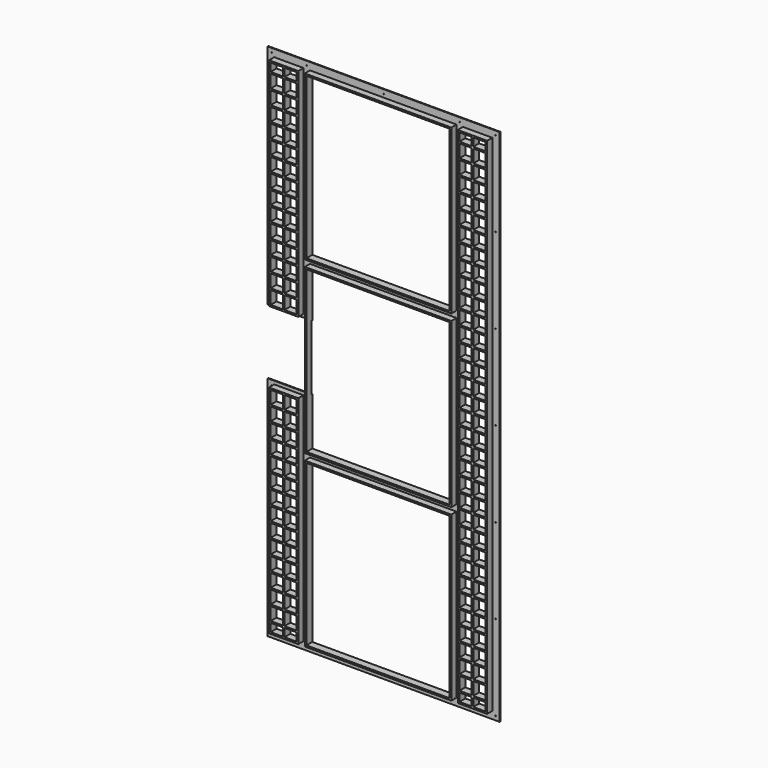
from build123d import *

# Parameters (mm, degrees)
F0_W      = 114.3
F0_H      = 844.55
F0_H_2    = 1968.5
F0_W_2    = 571.5
F0_H_3    = 25.4
F1_DEPTH  = 3.175
F2_W      = 114.3
F2_H      = 1968.5
F2_W_2    = 101.6000261307
F2_H_2    = 1955.8000261307
F2_W_3    = 571.5
F2_H_3    = 638.96875
F2_W_4    = 558.8
F2_H_4    = 626.26875
F2_H_5    = 639.7625
F2_H_6    = 627.0625
F2_H_7    = 844.55
F2_W_5    = 101.6000169754
F2_H_8    = 831.8500169754
F2_W_6    = 101.5999731064
F2_H_9    = 831.8499731064
F2_W_7    = 558.8000261307
F2_H_10   = 626.2687761307
F3_DEPTH  = 28.575
F4_W      = 47.6250084877
F4_H      = 6.35
F4_W_2    = 6.35
F4_H_2    = 50.8
F4_H_3    = 6.3500062943
F4_H_4    = 6.3500309944
F4_H_5    = 31.75
F4_H_6    = 6.3500188828
F4_H_7    = 6.3500125885
F5_DEPTH  = 28.575
F4_H_8    = 6.3500052452
F4_W_3    = 47.6249865532
F4_H_9    = 6.3499976873
F4_H_10   = 6.3499988437
F4_H_11   = 6.349999775
F4_H_12   = 6.349996756
F4_H_13   = 31.7498180389
F6_DEPTH  = 28.575
F4_H_14   = 31.7500045776
F4_W_4    = 47.6250130653
F7_DEPTH  = 28.575
F4_H_15   = 31.7498445511
F8_DEPTH  = 28.575
F9_DEPTH  = 28.575
F10_R     = 1.5875
F11_DEPTH = 25.4
F10_R_2   = 4.7625
F12_DEPTH = 1.5875
F13_W     = 19.05
F13_H     = 254
F14_DEPTH = 3.175


# Not quite as in the source:
# - ends of sketch curves that miss each other by under 0.0002 mm in the source are joined


with BuildPart() as f1:
    # F0 (on Front) → F1 (new body)
    with BuildSketch(Plane.XZ):
        Polygon((-450.85, -1508.125), (450.85, -1508.125), (450.85, 511.175), (-450.85, 511.175), (-450.85, -371.475), (-298.45, -371.475), (-298.45, -625.475), (-450.85, -625.475), align=None)
        with Locations((-368.3, -1060.45)):
            Rectangle(F0_W, F0_H, mode=Mode.SUBTRACT)
        Polygon((-285.75, -153.19375), (-285.75, 485.775), (285.75, 485.775), (285.75, -153.19375), (285.75, -178.59375), (285.75, -818.35625), (285.75, -843.75625), (285.75, -1482.725), (-285.75, -1482.725), (-285.75, -843.75625), (-285.75, -818.35625), (-285.75, -178.59375), align=None, mode=Mode.SUBTRACT)
        with Locations((-368.3, 63.5)):
            Rectangle(F0_W, F0_H, mode=Mode.SUBTRACT)
        with Locations((368.3, -498.475)):
            Rectangle(F0_W, F0_H_2, mode=Mode.SUBTRACT)
        Polygon((450.85, 511.175), (450.85, -1508.125), (-450.85, -1508.125), (-450.8499999999, -1511.3), (454.025, -1511.3), (454.025, 514.35), (-450.85, 514.35), (-450.85, 511.175), align=None)
        with Locations((0, -831.05625)):
            Rectangle(F0_W_2, F0_H_3)
        with Locations((0, -165.89375)):
            Rectangle(F0_W_2, F0_H_3)
    extrude(amount=F1_DEPTH)

    # F2 (on Front) → F3 (join)
    with BuildSketch(Plane.XZ):
        with Locations((368.3, -498.475)):
            Rectangle(F2_W, F2_H)
        with Locations((368.3, -498.475)):
            Rectangle(F2_W_2, F2_H_2, mode=Mode.SUBTRACT)
        with Locations((0, -1163.240625)):
            Rectangle(F2_W_3, F2_H_3)
        with Locations((0, -1163.240625)):
            Rectangle(F2_W_4, F2_H_4, mode=Mode.SUBTRACT)
        with Locations((0, -498.475)):
            Rectangle(F2_W_3, F2_H_5)
        with Locations((0, -498.475)):
            Rectangle(F2_W_4, F2_H_6, mode=Mode.SUBTRACT)
        with Locations((-368.3, -1060.45)):
            Rectangle(F2_W, F2_H_7)
        with Locations((-368.3, -1060.45)):
            Rectangle(F2_W_5, F2_H_8, mode=Mode.SUBTRACT)
        with Locations((-368.3, 63.5)):
            Rectangle(F2_W, F2_H_7)
        with Locations((-368.3, 63.5)):
            Rectangle(F2_W_6, F2_H_9, mode=Mode.SUBTRACT)
        with Locations((0, 166.290625)):
            Rectangle(F2_W_3, F2_H_3)
        with Locations((0, 166.290625)):
            Rectangle(F2_W_7, F2_H_10, mode=Mode.SUBTRACT)
    extrude(amount=F3_DEPTH)

    # F4 (on Front) → F5 (join)
    with BuildSketch(Plane.XZ):
        with Locations((-341.3124957561, -1098.5499523163)):
            Rectangle(F4_W, F4_H)
        with Locations((-368.3, -1098.5499523163)):
            Rectangle(F4_W_2, F4_H)
        with Locations((-395.2875042439, -1098.5499523163)):
            Rectangle(F4_W, F4_H)
        with Locations((-368.3, -1127.1249523163)):
            Rectangle(F4_W_2, F4_H_2)
        with Locations((-395.2875042439, -1155.6999523163)):
            Rectangle(F4_W, F4_H)
        with Locations((-368.3, -1155.6999523163)):
            Rectangle(F4_W_2, F4_H)
        with Locations((-341.3124957561, -1155.6999523163)):
            Rectangle(F4_W, F4_H)
        with Locations((-395.2875042439, -1212.8499554634)):
            Rectangle(F4_W, F4_H_3)
        with Locations((-368.3, -1212.8499554634)):
            Rectangle(F4_W_2, F4_H_3)
        with Locations((-341.3124957561, -1212.8499554634)):
            Rectangle(F4_W, F4_H_3)
        with Locations((-368.3, -1241.4249586105)):
            Rectangle(F4_W_2, F4_H_2)
        with Locations((-368.3, -1269.9999617577)):
            Rectangle(F4_W_2, F4_H_3)
        with Locations((-395.2875042439, -1269.9999617577)):
            Rectangle(F4_W, F4_H_3)
        with Locations((-341.3124957561, -1269.9999617577)):
            Rectangle(F4_W, F4_H_3)
        Polygon((-317.4999915123, -1330.324971199), (-317.4999915123, -1323.9749649048), (-365.125, -1323.9749649048), (-371.475, -1323.9749649048), (-419.1000084877, -1323.9749649048), (-419.1000084877, -1330.324971199), (-371.475, -1330.324971199), (-365.125, -1330.324971199), align=None)
        with Locations((-368.3, -1355.724971199)):
            Rectangle(F4_W_2, F4_H_2)
        Polygon((-317.4999915123, -1387.4749774933), (-317.4999915123, -1381.124971199), (-365.125, -1381.124971199), (-371.475, -1381.124971199), (-419.1000084877, -1381.124971199), (-419.1000084877, -1387.4749774933), (-371.475, -1387.4749774933), (-365.125, -1387.4749774933), align=None)
        with Locations((-395.2875042439, -1441.4499929905)):
            Rectangle(F4_W, F4_H_4)
        with Locations((-341.3124957561, -1441.4499929905)):
            Rectangle(F4_W, F4_H_4)
        with Locations((-368.3, -1441.4499929905)):
            Rectangle(F4_W_2, F4_H_4)
        with Locations((-368.3, -1460.5000084877)):
            Rectangle(F4_W_2, F4_H_5)
        with Locations((-368.3, -1041.3999428749)):
            Rectangle(F4_W_2, F4_H_6)
        with Locations((-395.2875042439, -1041.3999428749)):
            Rectangle(F4_W, F4_H_6)
        with Locations((-341.3124957561, -1041.3999428749)):
            Rectangle(F4_W, F4_H_6)
        with Locations((-368.3, -1012.8249334335)):
            Rectangle(F4_W_2, F4_H_2)
        with Locations((-395.2875042439, -984.2499302864)):
            Rectangle(F4_W, F4_H_3)
        with Locations((-368.3, -984.2499302864)):
            Rectangle(F4_W_2, F4_H_3)
        with Locations((-341.3124957561, -984.2499302864)):
            Rectangle(F4_W, F4_H_3)
        with Locations((-341.3124957561, -869.949920845)):
            Rectangle(F4_W, F4_H)
        with Locations((-395.2875042439, -869.949920845)):
            Rectangle(F4_W, F4_H)
        with Locations((-368.3, -869.949920845)):
            Rectangle(F4_W_2, F4_H)
        with Locations((-368.3, -927.0999239922)):
            Rectangle(F4_W_2, F4_H_3)
        with Locations((-341.3124957561, -927.0999239922)):
            Rectangle(F4_W, F4_H_3)
        with Locations((-368.3, -898.524920845)):
            Rectangle(F4_W_2, F4_H_2)
        with Locations((-395.2875042439, -927.0999239922)):
            Rectangle(F4_W, F4_H_3)
        with Locations((-368.3, -812.7999145508)):
            Rectangle(F4_W_2, F4_H_7)
        with Locations((-395.2875042439, -812.7999145508)):
            Rectangle(F4_W, F4_H_7)
        with Locations((-341.3124957561, -812.7999145508)):
            Rectangle(F4_W, F4_H_7)
        with Locations((-368.3, -784.2249082565)):
            Rectangle(F4_W_2, F4_H_2)
        with Locations((-368.3, -755.6499082565)):
            Rectangle(F4_W_2, F4_H)
        with Locations((-395.2875042439, -755.6499082565)):
            Rectangle(F4_W, F4_H)
        with Locations((-341.3124957561, -755.6499082565)):
            Rectangle(F4_W, F4_H)
        Polygon((-317.4999915123, -701.6749082565), (-317.4999915123, -695.324895668), (-365.125, -695.324895668), (-371.475, -695.324895668), (-419.1000084877, -695.324895668), (-419.1000084877, -701.6749082565), (-371.475, -701.6749082565), (-365.125, -701.6749082565), align=None)
        Polygon((-365.125, -695.324895668), (-365.125, -644.5249435902), (-371.475, -644.5249915123), (-371.475, -695.324895668), align=None)
    extrude(amount=F5_DEPTH)

    # F4 (on Front) → F6 (join)
    with BuildSketch(Plane.XZ):
        with Locations((-368.3, -327.0248589516)):
            Rectangle(F4_W_2, F4_H_2)
        with Locations((-368.3, -298.449856329)):
            Rectangle(F4_W_2, F4_H_8)
        Polygon((-371.475, -301.6248589516), (-371.475, -295.2748537064), (-419.1000084877, -295.2748537064), (-419.0999865532, -301.6248589516), align=None)
        with Locations((-341.3125067234, -298.449856329)):
            Rectangle(F4_W_3, F4_H_8)
        with Locations((-341.3125067234, -241.2998537064)):
            Rectangle(F4_W_3, F4_H)
        with Locations((-368.3, -241.2998537064)):
            Rectangle(F4_W_2, F4_H)
        Polygon((-371.475, -244.4748537064), (-371.475, -238.1248537064), (-419.1000084877, -238.1248537064), (-419.0999865532, -244.4748537064), align=None)
        with Locations((-368.3, -212.7248537064)):
            Rectangle(F4_W_2, F4_H_2)
        with Locations((-368.3, -184.1498548627)):
            Rectangle(F4_W_2, F4_H_9)
        with Locations((-395.2875042439, -184.1498548627)):
            Rectangle(F4_W, F4_H_9)
        with Locations((-341.3125067234, -184.1498548627)):
            Rectangle(F4_W_3, F4_H_9)
        with Locations((-395.2875042439, -126.9998565972)):
            Rectangle(F4_W, F4_H_10)
        with Locations((-341.3125067234, -126.9998565972)):
            Rectangle(F4_W_3, F4_H_10)
        with Locations((-368.3, -98.4248571754)):
            Rectangle(F4_W_2, F4_H_2)
        with Locations((-368.3, -126.9998565972)):
            Rectangle(F4_W_2, F4_H_10)
        with Locations((-368.3, -69.8498577535)):
            Rectangle(F4_W_2, F4_H_10)
        with Locations((-395.2875042439, -69.8498577535)):
            Rectangle(F4_W, F4_H_10)
        with Locations((-341.3125067234, -69.8498577535)):
            Rectangle(F4_W_3, F4_H_10)
        with Locations((-395.2875042439, -12.6998584442)):
            Rectangle(F4_W, F4_H_11)
        with Locations((-368.3, -12.6998584442)):
            Rectangle(F4_W_2, F4_H_11)
        with Locations((-341.3125067234, -12.6998584442)):
            Rectangle(F4_W_3, F4_H_11)
        with Locations((-368.3, 15.8751414433)):
            Rectangle(F4_W_2, F4_H_2)
        with Locations((-368.3, 44.4501414433)):
            Rectangle(F4_W_2, F4_H)
        with Locations((-395.2875042439, 44.4501414433)):
            Rectangle(F4_W, F4_H)
        with Locations((-341.3125067234, 44.4501414433)):
            Rectangle(F4_W_3, F4_H)
        with Locations((-395.2875042439, 101.6001398213)):
            Rectangle(F4_W, F4_H_12)
        with Locations((-368.3, 101.6001398213)):
            Rectangle(F4_W_2, F4_H_12)
        with Locations((-341.3125067234, 101.6001398213)):
            Rectangle(F4_W_3, F4_H_12)
        with Locations((-368.3, 130.1751381993)):
            Rectangle(F4_W_2, F4_H_2)
        with Locations((-368.3, 158.7501376212)):
            Rectangle(F4_W_2, F4_H_10)
        with Locations((-395.2875042439, 158.7501376212)):
            Rectangle(F4_W, F4_H_10)
        with Locations((-341.3125067234, 158.7501376212)):
            Rectangle(F4_W_3, F4_H_10)
        with Locations((-368.3, 215.9001401901)):
            Rectangle(F4_W_2, F4_H_3)
        with Locations((-395.2875042439, 215.9001401901)):
            Rectangle(F4_W, F4_H_3)
        with Locations((-341.3125067234, 215.9001401901)):
            Rectangle(F4_W_3, F4_H_3)
        with Locations((-368.3, 244.4751433372)):
            Rectangle(F4_W_2, F4_H_2)
        with Locations((-368.3, 273.0501464844)):
            Rectangle(F4_W_2, F4_H_3)
        with Locations((-395.2875042439, 273.0501464844)):
            Rectangle(F4_W, F4_H_3)
        with Locations((-341.3125067234, 273.0501464844)):
            Rectangle(F4_W_3, F4_H_3)
        with Locations((-368.3, 330.2001527786)):
            Rectangle(F4_W_2, F4_H_3)
        with Locations((-395.2875042439, 330.2001527786)):
            Rectangle(F4_W, F4_H_3)
        with Locations((-341.3125067234, 330.2001527786)):
            Rectangle(F4_W_3, F4_H_3)
        with Locations((-368.3, 358.7751559258)):
            Rectangle(F4_W_2, F4_H_2)
        with Locations((-368.3, 387.3501590729)):
            Rectangle(F4_W_2, F4_H_3)
        with Locations((-395.2875042439, 387.3501590729)):
            Rectangle(F4_W, F4_H_3)
        with Locations((-341.3125067234, 387.3501590729)):
            Rectangle(F4_W_3, F4_H_3)
        with Locations((-395.2875042439, 444.5001653671)):
            Rectangle(F4_W, F4_H_3)
        with Locations((-368.3, 444.5001653671)):
            Rectangle(F4_W_2, F4_H_3)
        with Locations((-341.3125067234, 444.5001653671)):
            Rectangle(F4_W_3, F4_H_3)
        with Locations((-368.3, 463.5500775337)):
            Rectangle(F4_W_2, F4_H_13)
    extrude(amount=F6_DEPTH)

    # F4 (on Front) → F7 (join)
    with BuildSketch(Plane.XZ):
        with Locations((368.3, -1460.5000107765)):
            Rectangle(F4_W_2, F4_H_14)
        with Locations((368.3, -1441.4499929905)):
            Rectangle(F4_W_2, F4_H_4)
        with Locations((341.3124934673, -1441.4499929905)):
            Rectangle(F4_W_4, F4_H_4)
        with Locations((395.2875065327, -1441.4499929905)):
            Rectangle(F4_W_4, F4_H_4)
        with Locations((368.3, -1384.2999743462)):
            Rectangle(F4_W_2, F4_H_3)
        with Locations((341.3124934673, -1384.2999743462)):
            Rectangle(F4_W_4, F4_H_3)
        with Locations((395.2875065327, -1384.2999743462)):
            Rectangle(F4_W_4, F4_H_3)
        with Locations((368.3, -1355.724971199)):
            Rectangle(F4_W_2, F4_H_2)
        with Locations((341.3124934673, -1327.1499680519)):
            Rectangle(F4_W_4, F4_H_3)
        with Locations((368.3, -1327.1499680519)):
            Rectangle(F4_W_2, F4_H_3)
        with Locations((395.2875065327, -1327.1499680519)):
            Rectangle(F4_W_4, F4_H_3)
        with Locations((368.3, -1269.9999617577)):
            Rectangle(F4_W_2, F4_H_3)
        with Locations((341.3124934673, -1269.9999617577)):
            Rectangle(F4_W_4, F4_H_3)
        with Locations((395.2875065327, -1269.9999617577)):
            Rectangle(F4_W_4, F4_H_3)
        with Locations((368.3, -1241.4249586105)):
            Rectangle(F4_W_2, F4_H_2)
        with Locations((368.3, -1212.8499554634)):
            Rectangle(F4_W_2, F4_H_3)
        with Locations((341.3124934673, -1212.8499554634)):
            Rectangle(F4_W_4, F4_H_3)
        with Locations((395.2875065327, -1212.8499554634)):
            Rectangle(F4_W_4, F4_H_3)
        with Locations((368.3, -1127.1249523163)):
            Rectangle(F4_W_2, F4_H_2)
        with Locations((368.3, -1098.5499523163)):
            Rectangle(F4_W_2, F4_H)
        with Locations((341.3124934673, -1098.5499523163)):
            Rectangle(F4_W_4, F4_H)
        with Locations((395.2875065327, -1098.5499523163)):
            Rectangle(F4_W_4, F4_H)
        with Locations((395.2875065327, -1155.6999523163)):
            Rectangle(F4_W_4, F4_H)
        with Locations((368.3, -1155.6999523163)):
            Rectangle(F4_W_2, F4_H)
        with Locations((341.3124934673, -1155.6999523163)):
            Rectangle(F4_W_4, F4_H)
        with Locations((341.3124934673, -1041.3999428749)):
            Rectangle(F4_W_4, F4_H_6)
        with Locations((395.2875065327, -1041.3999428749)):
            Rectangle(F4_W_4, F4_H_6)
        with Locations((368.3, -1041.3999428749)):
            Rectangle(F4_W_2, F4_H_6)
        with Locations((368.3, -1012.8249334335)):
            Rectangle(F4_W_2, F4_H_2)
        with Locations((368.3, -984.2499302864)):
            Rectangle(F4_W_2, F4_H_3)
        with Locations((341.3124934673, -984.2499302864)):
            Rectangle(F4_W_4, F4_H_3)
        with Locations((395.2875065327, -984.2499302864)):
            Rectangle(F4_W_4, F4_H_3)
        with Locations((368.3, -927.0999239922)):
            Rectangle(F4_W_2, F4_H_3)
        with Locations((341.3124934673, -927.0999239922)):
            Rectangle(F4_W_4, F4_H_3)
        with Locations((368.3, -898.524920845)):
            Rectangle(F4_W_2, F4_H_2)
        with Locations((395.2875065327, -927.0999239922)):
            Rectangle(F4_W_4, F4_H_3)
        with Locations((368.3, -869.949920845)):
            Rectangle(F4_W_2, F4_H)
        with Locations((395.2875065327, -869.949920845)):
            Rectangle(F4_W_4, F4_H)
        with Locations((341.3124934673, -869.949920845)):
            Rectangle(F4_W_4, F4_H)
        with Locations((341.3124934673, -812.7999145508)):
            Rectangle(F4_W_4, F4_H_7)
        with Locations((395.2875065327, -812.7999145508)):
            Rectangle(F4_W_4, F4_H_7)
        with Locations((368.3, -755.6499082565)):
            Rectangle(F4_W_2, F4_H)
        with Locations((341.3124934673, -755.6499082565)):
            Rectangle(F4_W_4, F4_H)
        with Locations((395.2875065327, -755.6499082565)):
            Rectangle(F4_W_4, F4_H)
        with Locations((368.3, -784.2249082565)):
            Rectangle(F4_W_2, F4_H_2)
        with Locations((368.3, -812.7999145508)):
            Rectangle(F4_W_2, F4_H_7)
        with Locations((368.3, -698.4999019623)):
            Rectangle(F4_W_2, F4_H_7)
        with Locations((341.3124934673, -698.4999019623)):
            Rectangle(F4_W_4, F4_H_7)
        with Locations((395.2875065327, -698.4999019623)):
            Rectangle(F4_W_4, F4_H_7)
        with Locations((368.3, -669.924895668)):
            Rectangle(F4_W_2, F4_H_2)
        with Locations((368.3, -641.3498930454)):
            Rectangle(F4_W_2, F4_H_8)
        with Locations((341.3124934673, -641.3498930454)):
            Rectangle(F4_W_4, F4_H_8)
        with Locations((395.2875065327, -641.3498930454)):
            Rectangle(F4_W_4, F4_H_8)
        with Locations((368.3, -584.1998904228)):
            Rectangle(F4_W_2, F4_H)
        with Locations((395.2875065327, -584.1998904228)):
            Rectangle(F4_W_4, F4_H)
        with Locations((368.3, -555.6248904228)):
            Rectangle(F4_W_2, F4_H_2)
        with Locations((368.3, -527.0498841286)):
            Rectangle(F4_W_2, F4_H_7)
        with Locations((341.3124934673, -527.0498841286)):
            Rectangle(F4_W_4, F4_H_7)
        with Locations((395.2875065327, -527.0498841286)):
            Rectangle(F4_W_4, F4_H_7)
        with Locations((341.3124934673, -584.1998904228)):
            Rectangle(F4_W_4, F4_H)
        with Locations((341.3124934673, -469.8998746872)):
            Rectangle(F4_W_4, F4_H_3)
        with Locations((395.2875065327, -469.8998746872)):
            Rectangle(F4_W_4, F4_H_3)
        with Locations((368.3, -441.3248715401)):
            Rectangle(F4_W_2, F4_H_2)
        with Locations((368.3, -469.8998746872)):
            Rectangle(F4_W_2, F4_H_3)
        with Locations((395.2875065327, -412.7498683929)):
            Rectangle(F4_W_4, F4_H_3)
        with Locations((341.3124934673, -412.7498683929)):
            Rectangle(F4_W_4, F4_H_3)
        with Locations((368.3, -412.7498683929)):
            Rectangle(F4_W_2, F4_H_3)
        with Locations((368.3, -355.5998620987)):
            Rectangle(F4_W_2, F4_H_3)
        with Locations((341.3124934673, -355.5998620987)):
            Rectangle(F4_W_4, F4_H_3)
        with Locations((395.2875065327, -355.5998620987)):
            Rectangle(F4_W_4, F4_H_3)
        with Locations((368.3, -327.0248589516)):
            Rectangle(F4_W_2, F4_H_2)
        with Locations((368.3, -298.449856329)):
            Rectangle(F4_W_2, F4_H_8)
        with Locations((341.3124934673, -298.449856329)):
            Rectangle(F4_W_4, F4_H_8)
        with Locations((395.2875065327, -298.449856329)):
            Rectangle(F4_W_4, F4_H_8)
        with Locations((368.3, -241.2998537064)):
            Rectangle(F4_W_2, F4_H)
        with Locations((341.3124934673, -241.2998537064)):
            Rectangle(F4_W_4, F4_H)
        with Locations((395.2875065327, -241.2998537064)):
            Rectangle(F4_W_4, F4_H)
        with Locations((368.3, -212.7248537064)):
            Rectangle(F4_W_2, F4_H_2)
        with Locations((368.3, -184.1498548627)):
            Rectangle(F4_W_2, F4_H_9)
        with Locations((341.3124934673, -184.1498548627)):
            Rectangle(F4_W_4, F4_H_9)
        with Locations((395.2875065327, -184.1498548627)):
            Rectangle(F4_W_4, F4_H_9)
        with Locations((368.3, -126.9998565972)):
            Rectangle(F4_W_2, F4_H_10)
        with Locations((341.3124934673, -126.9998565972)):
            Rectangle(F4_W_4, F4_H_10)
        with Locations((395.2875065327, -126.9998565972)):
            Rectangle(F4_W_4, F4_H_10)
        with Locations((368.3, -98.4248571753)):
            Rectangle(F4_W_2, F4_H_2)
        with Locations((368.3, -69.8498577535)):
            Rectangle(F4_W_2, F4_H_10)
        with Locations((395.2875065327, -69.8498577535)):
            Rectangle(F4_W_4, F4_H_10)
        with Locations((341.3124934673, -69.8498577535)):
            Rectangle(F4_W_4, F4_H_10)
    extrude(amount=F7_DEPTH)

    # F4 (on Front) → F8 (join)
    with BuildSketch(Plane.XZ):
        with Locations((368.3, -12.6998584442)):
            Rectangle(F4_W_2, F4_H_11)
        with Locations((341.3124934673, -12.6998584442)):
            Rectangle(F4_W_4, F4_H_11)
        with Locations((395.2875065327, -12.6998584442)):
            Rectangle(F4_W_4, F4_H_11)
        with Locations((368.3, 15.8751414433)):
            Rectangle(F4_W_2, F4_H_2)
        with Locations((368.3, 44.4501414433)):
            Rectangle(F4_W_2, F4_H)
        with Locations((341.3124934673, 44.4501414433)):
            Rectangle(F4_W_4, F4_H)
        with Locations((395.2875065327, 44.4501414433)):
            Rectangle(F4_W_4, F4_H)
        with Locations((368.3, 101.6001398213)):
            Rectangle(F4_W_2, F4_H_12)
        with Locations((341.3124934673, 101.6001398213)):
            Rectangle(F4_W_4, F4_H_12)
        with Locations((395.2875065327, 101.6001398213)):
            Rectangle(F4_W_4, F4_H_12)
        with Locations((368.3, 130.1751381993)):
            Rectangle(F4_W_2, F4_H_2)
        with Locations((368.3, 158.7501376212)):
            Rectangle(F4_W_2, F4_H_10)
        with Locations((341.3124934673, 158.7501376212)):
            Rectangle(F4_W_4, F4_H_10)
        with Locations((395.2875065327, 158.7501376212)):
            Rectangle(F4_W_4, F4_H_10)
        with Locations((368.3, 215.9001401901)):
            Rectangle(F4_W_2, F4_H_3)
        with Locations((341.3124934673, 215.9001401901)):
            Rectangle(F4_W_4, F4_H_3)
        with Locations((368.3, 244.4751433373)):
            Rectangle(F4_W_2, F4_H_2)
        with Locations((395.2875065327, 215.9001401901)):
            Rectangle(F4_W_4, F4_H_3)
        with Locations((368.3, 273.0501464844)):
            Rectangle(F4_W_2, F4_H_3)
        with Locations((341.3124934673, 273.0501464844)):
            Rectangle(F4_W_4, F4_H_3)
        with Locations((395.2875065327, 273.0501464844)):
            Rectangle(F4_W_4, F4_H_3)
        with Locations((368.3, 330.2001527786)):
            Rectangle(F4_W_2, F4_H_3)
        with Locations((341.3124934673, 330.2001527786)):
            Rectangle(F4_W_4, F4_H_3)
        with Locations((395.2875065327, 330.2001527786)):
            Rectangle(F4_W_4, F4_H_3)
        with Locations((368.3, 358.7751559258)):
            Rectangle(F4_W_2, F4_H_2)
        with Locations((368.3, 387.3501590729)):
            Rectangle(F4_W_2, F4_H_3)
        with Locations((341.3124934673, 387.3501590729)):
            Rectangle(F4_W_4, F4_H_3)
        with Locations((395.2875065327, 387.3501590729)):
            Rectangle(F4_W_4, F4_H_3)
        with Locations((368.3, 463.5500907898)):
            Rectangle(F4_W_2, F4_H_15)
        with Locations((368.3, 444.5001653671)):
            Rectangle(F4_W_2, F4_H_3)
        with Locations((341.3124934673, 444.5001653671)):
            Rectangle(F4_W_4, F4_H_3)
        with Locations((395.2875065327, 444.5001653671)):
            Rectangle(F4_W_4, F4_H_3)
    extrude(amount=F8_DEPTH)

    # F4 (on Front) → F9 (join)
    with BuildSketch(Plane.XZ):
        with Locations((-368.3, -1412.8749774933)):
            Rectangle(F4_W_2, F4_H_2)
        with Locations((-368.3, -1298.5749649048)):
            Rectangle(F4_W_2, F4_H_2)
        with Locations((-368.3, -1184.2749523163)):
            Rectangle(F4_W_2, F4_H_2)
        with Locations((-368.3, -1069.9749523163)):
            Rectangle(F4_W_2, F4_H_2)
        with Locations((-368.3, -955.6749271393)):
            Rectangle(F4_W_2, F4_H_2)
        with Locations((-368.3, -841.374920845)):
            Rectangle(F4_W_2, F4_H_2)
        with Locations((-368.3, -727.0749082565)):
            Rectangle(F4_W_2, F4_H_2)
        with Locations((368.3, -1412.8749774933)):
            Rectangle(F4_W_2, F4_H_2)
        with Locations((368.3, -1298.5749649048)):
            Rectangle(F4_W_2, F4_H_2)
        with Locations((368.3, -1184.2749523163)):
            Rectangle(F4_W_2, F4_H_2)
        with Locations((368.3, -1069.9749523163)):
            Rectangle(F4_W_2, F4_H_2)
        with Locations((368.3, -955.6749271393)):
            Rectangle(F4_W_2, F4_H_2)
        with Locations((368.3, -841.374920845)):
            Rectangle(F4_W_2, F4_H_2)
        with Locations((368.3, -727.0749082565)):
            Rectangle(F4_W_2, F4_H_2)
        with Locations((368.3, -612.7748904228)):
            Rectangle(F4_W_2, F4_H_2)
        with Locations((368.3, -498.4748778343)):
            Rectangle(F4_W_2, F4_H_2)
        with Locations((368.3, -269.8748537064)):
            Rectangle(F4_W_2, F4_H_2)
        with Locations((368.3, -384.1748652458)):
            Rectangle(F4_W_2, F4_H_2)
        with Locations((368.3, -41.2748583317)):
            Rectangle(F4_W_2, F4_H_2)
        with Locations((368.3, 73.0251414433)):
            Rectangle(F4_W_2, F4_H_2)
        with Locations((368.3, -155.574856019)):
            Rectangle(F4_W_2, F4_H_2)
        with Locations((368.3, 187.325137043)):
            Rectangle(F4_W_2, F4_H_2)
        with Locations((368.3, 301.6251496315)):
            Rectangle(F4_W_2, F4_H_2)
        with Locations((368.3, 415.92516222)):
            Rectangle(F4_W_2, F4_H_2)
        with Locations((-368.3, 415.92516222)):
            Rectangle(F4_W_2, F4_H_2)
        with Locations((-368.3, 301.6251496315)):
            Rectangle(F4_W_2, F4_H_2)
        with Locations((-368.3, 187.325137043)):
            Rectangle(F4_W_2, F4_H_2)
        with Locations((-368.3, 73.0251414433)):
            Rectangle(F4_W_2, F4_H_2)
        with Locations((-368.3, -41.2748583317)):
            Rectangle(F4_W_2, F4_H_2)
        with Locations((-368.3, -155.574856019)):
            Rectangle(F4_W_2, F4_H_2)
        with Locations((-368.3, -269.8748537064)):
            Rectangle(F4_W_2, F4_H_2)
    extrude(amount=F9_DEPTH)

    # F10 (on face) → F11 (cut)
    with BuildSketch(Plane(origin=(0, 0, 0), x_dir=(-1, 0, 0), z_dir=(0, 1, 0))):
        with Locations((-298.4499934673, 166.290625)):
            Circle(F10_R)
        with Locations((-438.15, 166.290625)):
            Circle(F10_R)
        with Locations((-298.4499934673, -165.8937630653)):
            Circle(F10_R)
        with Locations((-438.15, -165.8937630653)):
            Circle(F10_R)
        with Locations((-438.15, -498.475)):
            Circle(F10_R)
        with Locations((-298.4499934673, -498.4749967337)):
            Circle(F10_R)
        with Locations((-438.15, -831.05625)):
            Circle(F10_R)
        with Locations((-298.4499934673, -831.05625)):
            Circle(F10_R)
        with Locations((-438.15, -1163.240625)):
            Circle(F10_R)
        with Locations((-298.4499934673, -1163.240625)):
            Circle(F10_R)
        with Locations((-438.15, -1495.4250130653)):
            Circle(F10_R)
        with Locations((-298.4499934673, -1495.4250130653)):
            Circle(F10_R)
        with Locations((-1.5874999998, -1495.4250130653)):
            Circle(F10_R)
        with Locations((298.45, -1495.4250130653)):
            Circle(F10_R)
        with Locations((434.9750000004, -1495.4250130653)):
            Circle(F10_R)
        with Locations((298.45, -1163.240625)):
            Circle(F10_R)
        with Locations((434.9750000004, -1163.240625)):
            Circle(F10_R)
        with Locations((298.45, -831.05625)):
            Circle(F10_R)
        with Locations((434.9750000004, -831.05625)):
            Circle(F10_R)
        with Locations((0, -831.05625)):
            Circle(F10_R)
        with Locations((298.45, -644.5249915123)):
            Circle(F10_R)
        with Locations((434.9750000004, -644.5249915123)):
            Circle(F10_R)
        with Locations((298.45, -352.4249865532)):
            Circle(F10_R)
        with Locations((434.975, -352.4248589516)):
            Circle(F10_R)
        with Locations((434.975, -165.8937630653)):
            Circle(F10_R)
        with Locations((298.4500130653, -165.8937630653)):
            Circle(F10_R)
        with Locations((9.799e-06, -165.8937630653)):
            Circle(F10_R)
        with Locations((298.4500130653, 166.290625)):
            Circle(F10_R)
        with Locations((434.975, 166.290625)):
            Circle(F10_R)
        with Locations((298.4500130653, 498.4749906987)):
            Circle(F10_R)
        with Locations((434.975, 498.4749865532)):
            Circle(F10_R)
        with Locations((-1.5875, 498.4749998093)):
            Circle(F10_R)
        with Locations((-298.4499934673, 498.4750088234)):
            Circle(F10_R)
        with Locations((-438.15, 498.4750130653)):
            Circle(F10_R)
    extrude(amount=-F11_DEPTH, mode=Mode.SUBTRACT)

    # F10 (on face) → F12 (cut)
    with BuildSketch(Plane(origin=(0, 0, 0), x_dir=(-1, 0, 0), z_dir=(0, 1, 0))):
        with Locations((-298.4499934673, 498.4750088234)):
            Circle(F10_R_2)
        with Locations((-298.4499934673, 498.4750088234)):
            Circle(F10_R, mode=Mode.SUBTRACT)
        with Locations((-1.5875, 498.4749998093)):
            Circle(F10_R_2)
        with Locations((-1.5875, 498.4749998093)):
            Circle(F10_R, mode=Mode.SUBTRACT)
        with Locations((298.4500130653, 498.4749906987)):
            Circle(F10_R_2)
        with Locations((298.4500130653, 498.4749906987)):
            Circle(F10_R, mode=Mode.SUBTRACT)
        with Locations((434.975, 498.4749865532)):
            Circle(F10_R_2)
        with Locations((434.975, 498.4749865532)):
            Circle(F10_R, mode=Mode.SUBTRACT)
        with Locations((298.4500130653, 166.290625)):
            Circle(F10_R_2)
        with Locations((298.4500130653, 166.290625)):
            Circle(F10_R, mode=Mode.SUBTRACT)
        with Locations((434.975, 166.290625)):
            Circle(F10_R_2)
        with Locations((434.975, 166.290625)):
            Circle(F10_R, mode=Mode.SUBTRACT)
        with Locations((298.4500130653, -165.8937630653)):
            Circle(F10_R_2)
        with Locations((298.4500130653, -165.8937630653)):
            Circle(F10_R, mode=Mode.SUBTRACT)
        with Locations((434.975, -165.8937630653)):
            Circle(F10_R_2)
        with Locations((434.975, -165.8937630653)):
            Circle(F10_R, mode=Mode.SUBTRACT)
        with Locations((434.975, -352.4248589516)):
            Circle(F10_R_2)
        with Locations((434.975, -352.4248589516)):
            Circle(F10_R, mode=Mode.SUBTRACT)
        with Locations((298.45, -352.4249865532)):
            Circle(F10_R_2)
        with Locations((298.45, -352.4249865532)):
            Circle(F10_R, mode=Mode.SUBTRACT)
        with Locations((9.799e-06, -165.8937630653)):
            Circle(F10_R_2)
        with Locations((9.799e-06, -165.8937630653)):
            Circle(F10_R, mode=Mode.SUBTRACT)
        with Locations((-298.4499934673, -165.8937630653)):
            Circle(F10_R_2)
        with Locations((-298.4499934673, -165.8937630653)):
            Circle(F10_R, mode=Mode.SUBTRACT)
        with Locations((-438.15, -165.8937630653)):
            Circle(F10_R_2)
        with Locations((-438.15, -165.8937630653)):
            Circle(F10_R, mode=Mode.SUBTRACT)
        with Locations((-438.15, 166.290625)):
            Circle(F10_R_2)
        with Locations((-438.15, 166.290625)):
            Circle(F10_R, mode=Mode.SUBTRACT)
        with Locations((-298.4499934673, 166.290625)):
            Circle(F10_R_2)
        with Locations((-298.4499934673, 166.290625)):
            Circle(F10_R, mode=Mode.SUBTRACT)
        with Locations((-438.15, 498.4750130653)):
            Circle(F10_R_2)
        with Locations((-438.15, 498.4750130653)):
            Circle(F10_R, mode=Mode.SUBTRACT)
        with Locations((-298.4499934673, -498.4749967337)):
            Circle(F10_R_2)
        with Locations((-298.4499934673, -498.4749967337)):
            Circle(F10_R, mode=Mode.SUBTRACT)
        with Locations((-438.15, -498.475)):
            Circle(F10_R_2)
        with Locations((-438.15, -498.475)):
            Circle(F10_R, mode=Mode.SUBTRACT)
        with Locations((-438.15, -831.05625)):
            Circle(F10_R_2)
        with Locations((-438.15, -831.05625)):
            Circle(F10_R, mode=Mode.SUBTRACT)
        with Locations((-298.4499934673, -831.05625)):
            Circle(F10_R_2)
        with Locations((-298.4499934673, -831.05625)):
            Circle(F10_R, mode=Mode.SUBTRACT)
        with Locations((-298.4499934673, -1163.240625)):
            Circle(F10_R_2)
        with Locations((-298.4499934673, -1163.240625)):
            Circle(F10_R, mode=Mode.SUBTRACT)
        with Locations((-438.15, -1163.240625)):
            Circle(F10_R_2)
        with Locations((-438.15, -1163.240625)):
            Circle(F10_R, mode=Mode.SUBTRACT)
        with Locations((-438.15, -1495.4250130653)):
            Circle(F10_R_2)
        with Locations((-438.15, -1495.4250130653)):
            Circle(F10_R, mode=Mode.SUBTRACT)
        with Locations((-298.4499934673, -1495.4250130653)):
            Circle(F10_R_2)
        with Locations((-298.4499934673, -1495.4250130653)):
            Circle(F10_R, mode=Mode.SUBTRACT)
        with Locations((-1.5874999998, -1495.4250130653)):
            Circle(F10_R_2)
        with Locations((-1.5874999998, -1495.4250130653)):
            Circle(F10_R, mode=Mode.SUBTRACT)
        with Locations((298.45, -1495.4250130653)):
            Circle(F10_R_2)
        with Locations((298.45, -1495.4250130653)):
            Circle(F10_R, mode=Mode.SUBTRACT)
        with Locations((434.9750000004, -1495.4250130653)):
            Circle(F10_R_2)
        with Locations((434.9750000004, -1495.4250130653)):
            Circle(F10_R, mode=Mode.SUBTRACT)
        with Locations((298.45, -1163.240625)):
            Circle(F10_R_2)
        with Locations((298.45, -1163.240625)):
            Circle(F10_R, mode=Mode.SUBTRACT)
        with Locations((434.9750000004, -1163.240625)):
            Circle(F10_R_2)
        with Locations((434.9750000004, -1163.240625)):
            Circle(F10_R, mode=Mode.SUBTRACT)
        with Locations((0, -831.05625)):
            Circle(F10_R_2)
        with Locations((0, -831.05625)):
            Circle(F10_R, mode=Mode.SUBTRACT)
        with Locations((298.45, -831.05625)):
            Circle(F10_R_2)
        with Locations((298.45, -831.05625)):
            Circle(F10_R, mode=Mode.SUBTRACT)
        with Locations((434.9750000004, -831.05625)):
            Circle(F10_R_2)
        with Locations((434.9750000004, -831.05625)):
            Circle(F10_R, mode=Mode.SUBTRACT)
        with Locations((298.45, -644.5249915123)):
            Circle(F10_R_2)
        with Locations((298.45, -644.5249915123)):
            Circle(F10_R, mode=Mode.SUBTRACT)
        with Locations((434.9750000004, -644.5249915123)):
            Circle(F10_R_2)
        with Locations((434.9750000004, -644.5249915123)):
            Circle(F10_R, mode=Mode.SUBTRACT)
    extrude(amount=-F12_DEPTH, mode=Mode.SUBTRACT)

    # F13 (on face) → F14 (cut)
    with BuildSketch(Plane(origin=(0, 0, 0), x_dir=(-1, 0, 0), z_dir=(0, 1, 0))):
        with Locations((288.925, -498.475)):
            Rectangle(F13_W, F13_H)
    extrude(amount=-F14_DEPTH, mode=Mode.SUBTRACT)


solid = f1.part
